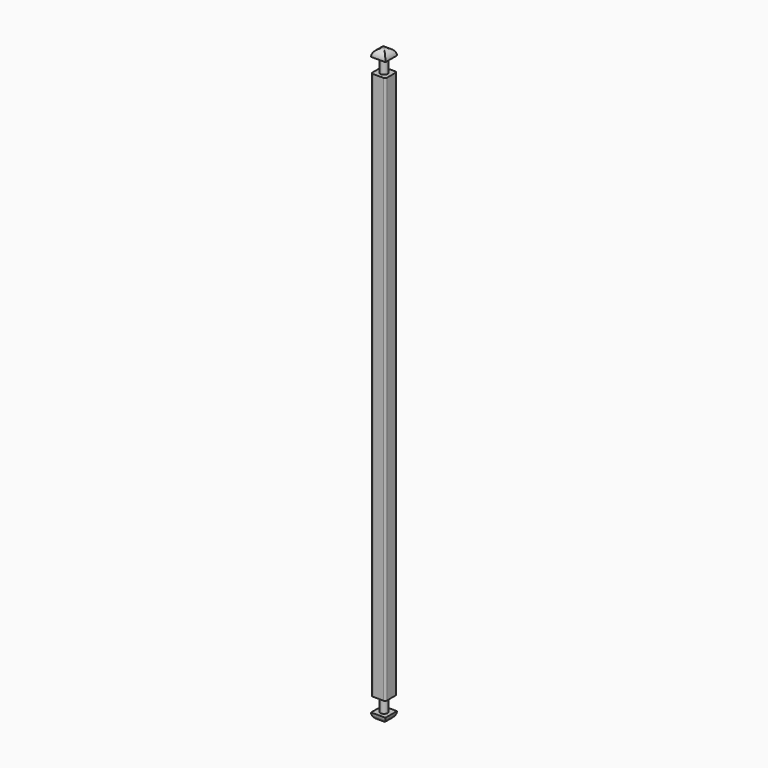
from build123d import *

# Parameters (mm, degrees)
F0_W      = 12.7
F0_H      = 12.7
F1_DEPTH  = 482.6
F2_R      = 3.175
F3_DEPTH  = 12.7
F4_R      = 3.175
F5_DEPTH  = 12.7
F6_W      = 12.7
F6_H      = 12.7
F7_DEPTH  = 6.35
F8_R      = 6.34999
F9_W      = 12.7
F9_H      = 12.7
F10_DEPTH = 6.35
F11_R     = 6.34999
F12_R     = 1.5875


# Not quite as in the source:
# - a fillet or chamfer is up to 0.001 mm smaller than in the source, because OpenCascade refuses the exact size


with BuildPart() as f1:
    # F0 (on Top) → F1 (new body)
    with BuildSketch(Plane.XY):
        with Locations((6.35, 6.35)):
            Rectangle(F0_W, F0_H)
    extrude(amount=-F1_DEPTH)

    # F2 (on face) → F3 (join)
    with BuildSketch(Plane.XY):
        with Locations((6.35, 6.35)):
            Circle(F2_R)
    extrude(amount=F3_DEPTH)

    # F4 (on face) → F5 (join)
    with BuildSketch(Plane(origin=(0, 0, -482.6), x_dir=(1, 0, 0), z_dir=(0, 0, -1))):
        with Locations((6.35, -6.35)):
            Circle(F4_R)
    extrude(amount=F5_DEPTH)

    # F6 (on face) → F7 (join)
    with BuildSketch(Plane.XY.offset(12.7)):
        with Locations((6.35, 6.35)):
            Rectangle(F6_W, F6_H)
    extrude(amount=F7_DEPTH)

    # F8 (radius 6.35 in the source; OpenCascade refuses exactly that, so slightly less here)
    f8_edges = [f1.edges().sort_by_distance(p)[0] for p in [
        (0, 6.35, 19.05),
        (6.35, 0, 19.05),
        (12.7, 6.35, 19.05),
        (6.35, 12.7, 19.05),
    ]]
    fillet(f8_edges, radius=F8_R)

    # F9 (on face) → F10 (join)
    with BuildSketch(Plane(origin=(0, 0, -495.3), x_dir=(1, 0, 0), z_dir=(0, 0, -1))):
        with Locations((6.35, -6.35)):
            Rectangle(F9_W, F9_H)
    extrude(amount=F10_DEPTH)

    # F11 (radius 6.35 in the source; OpenCascade refuses exactly that, so slightly less here)
    f11_edges = [f1.edges().sort_by_distance(p)[0] for p in [
        (6.35, 0, -501.65),
        (0, 6.35, -501.65),
        (6.35, 12.7, -501.65),
        (12.7, 6.35, -501.65),
    ]]
    fillet(f11_edges, radius=F11_R)

    # F12
    f12_edges = [f1.edges().sort_by_distance(p)[0] for p in [
        (0, 0, -241.3),
        (0, 12.7, -241.3),
        (12.7, 0, -241.3),
        (12.7, 12.7, -241.3),
    ]]
    fillet(f12_edges, radius=F12_R)


solid = f1.part
